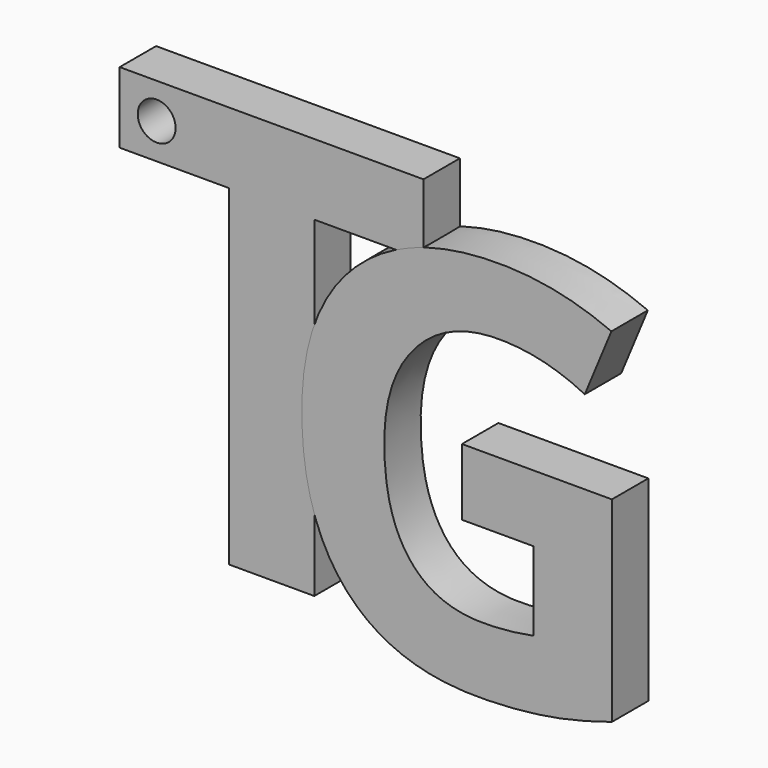
from build123d import *

# Parameters (mm, degrees)
F0_TEXT_SIZE = 37.1497848796
F1_DEPTH     = 3
F2_TEXT_SIZE = 34.8868547007
F3_DEPTH     = 3
F6_DEPTH     = 25


# Not quite as in the source:
# - Text() gives the source's letters only with a copy of the font that has no kerning and outlines rounded to 1/6400 em; it was checked with that copy


with BuildPart() as f1:
    # F0 (on Front) → F1 (new body)
    with BuildSketch(Plane.XZ):
        with Locations((-33.5366390646, 0)):
            Text('T', F0_TEXT_SIZE, font='Open Sans', font_style=FontStyle.BOLD, text_align=(TextAlign.LEFT, TextAlign.BOTTOM))
    extrude(amount=F1_DEPTH)

    # F5 (on face) → F6 (cut)
    with BuildSketch(Plane.XZ.offset(3)):
        with BuildLine():
            ThreePointArc((-31.605129391, 24.182188095), (-30.355129391, 22.932188095), (-29.105129391, 24.182188095))
            ThreePointArc((-29.105129391, 24.182188095), (-30.355129391, 25.432188095), (-31.605129391, 24.182188095))
        make_face()
    extrude(amount=-F6_DEPTH, mode=Mode.SUBTRACT)


with BuildPart() as f3:
    # F2 (on Front) → F3 (new body)
    with BuildSketch(Plane.XZ):
        with Locations((-62.3174746328, 0)):
            Text('G', F2_TEXT_SIZE, font='Open Sans', font_style=FontStyle.BOLD, text_align=(TextAlign.LEFT, TextAlign.BOTTOM))
    extrude(amount=F3_DEPTH)


with BuildPart() as f3_1:
    # F4: moved
    add(f3.part.moved(Location((39.5, 0, -2))))


solid = Compound([f1.part, f3_1.part])
